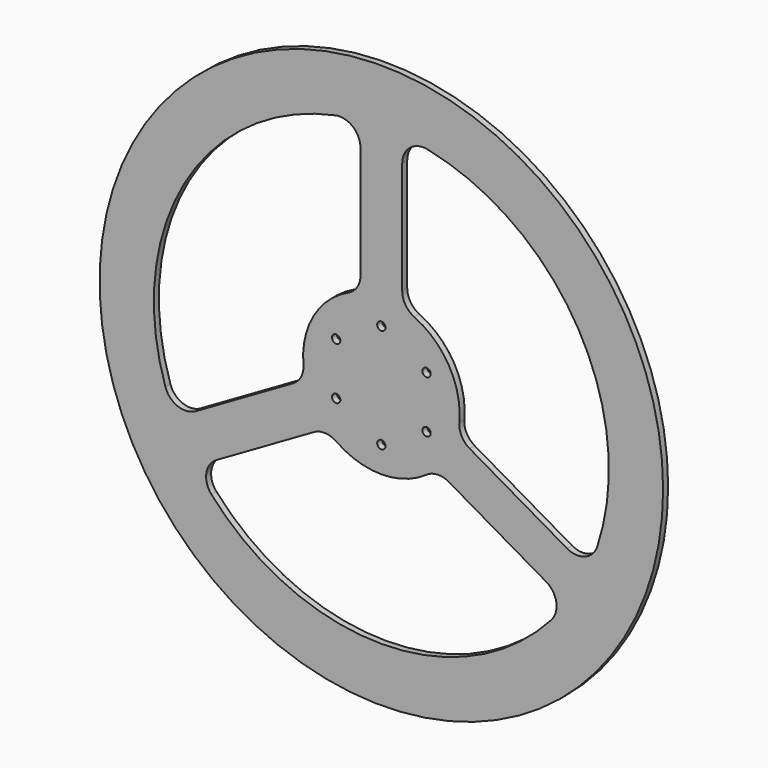
from build123d import *

# Parameters (mm, degrees)
F0_R            = 135
F1_DEPTH        = 3
F3_D            = 4
F3_COPIES_COUNT = 6


# Not quite as in the source:
# - a pattern or mirror of a feature is missing from the dataset's text; its kind, count and spacing are read off the source's solid


with BuildPart() as f1:
    # F0 (on Front) → F1 (new body)
    with BuildSketch(Plane.XZ):
        Circle(F0_R)
        with BuildLine():
            Line((-78.968744185, -57.1396310965), (-32.3120288915, -30.2023639624))
            ThreePointArc((-32.3120288915, -30.2023639624), (-26.8672094621, -28.8725161151), (-21.5621280722, -30.6810142107))
            ThreePointArc((-21.5621280722, -30.6810142107), (0, -37.5), (21.5621280722, -30.6810142107))
            ThreePointArc((21.5621280722, -30.6810142107), (26.8672094621, -28.8725161151), (32.3120288915, -30.2023639624))
            Line((32.3120288915, -30.2023639624), (78.968744185, -57.1396310965))
            ThreePointArc((78.968744185, -57.1396310965), (83.8408747407, -64.2058216819), (81.4403345067, -72.4463381783))
            ThreePointArc((81.4403345067, -72.4463381783), (0, -109), (-81.4403345067, -72.4463381783))
            ThreePointArc((-81.4403345067, -72.4463381783), (-83.8408747407, -64.2058216819), (-78.968744185, -57.1396310965))
        make_face(mode=Mode.SUBTRACT)
        with BuildLine():
            ThreePointArc((-10, 43.084219849), (-11.5707276958, 37.7039439805), (-15.7894736842, 34.0138577756))
            ThreePointArc((-15.7894736842, 34.0138577756), (-32.4759526419, 18.75), (-37.3516017564, -3.3328435649))
            ThreePointArc((-37.3516017564, -3.3328435649), (-38.4379371579, -8.8314278655), (-42.3120288915, -12.8818558867))
            Line((-42.3120288915, -12.8818558867), (-88.968744185, -39.8191230209))
            ThreePointArc((-88.968744185, -39.8191230209), (-97.5243100178, -40.50541656), (-103.4605365269, -34.3062294864))
            ThreePointArc((-103.4605365269, -34.3062294864), (-94.3967690125, 54.5), (-22.0202020202, 106.7525676646))
            ThreePointArc((-22.0202020202, 106.7525676646), (-13.6834352771, 104.7112382419), (-10, 96.9587541174))
            Line((-10, 96.9587541174), (-10, 43.084219849))
        make_face(mode=Mode.SUBTRACT)
        with BuildLine():
            ThreePointArc((15.7894736842, 34.0138577756), (11.5707276958, 37.7039439805), (10, 43.084219849))
            Line((10, 43.084219849), (10, 96.9587541174))
            ThreePointArc((10, 96.9587541174), (13.6834352771, 104.7112382419), (22.0202020202, 106.7525676646))
            ThreePointArc((22.0202020202, 106.7525676646), (94.3967690125, 54.5), (103.4605365269, -34.3062294864))
            ThreePointArc((103.4605365269, -34.3062294864), (97.5243100178, -40.50541656), (88.968744185, -39.8191230209))
            Line((88.968744185, -39.8191230209), (42.3120288915, -12.8818558867))
            ThreePointArc((42.3120288915, -12.8818558867), (38.4379371579, -8.8314278655), (37.3516017564, -3.3328435649))
            ThreePointArc((37.3516017564, -3.3328435649), (32.4759526419, 18.75), (15.7894736842, 34.0138577756))
        make_face(mode=Mode.SUBTRACT)
    extrude(amount=F1_DEPTH)

    # F3 (through all)
    with Locations(Plane(origin=(0, 0, 0), x_dir=(1, 0, 0), z_dir=(0, 1, 0))):
        with Locations((0, -25)):
            f3 = Hole(F3_D / 2)

    # F3_copies: F3 ×6 about axis
    f3_copies_axis = Axis((0, 0, 0), (0, 1, 0))
    for i in range(1, F3_COPIES_COUNT):
        add(f3.rotate(f3_copies_axis, i * 360 / F3_COPIES_COUNT), mode=Mode.SUBTRACT)


solid = f1.part
